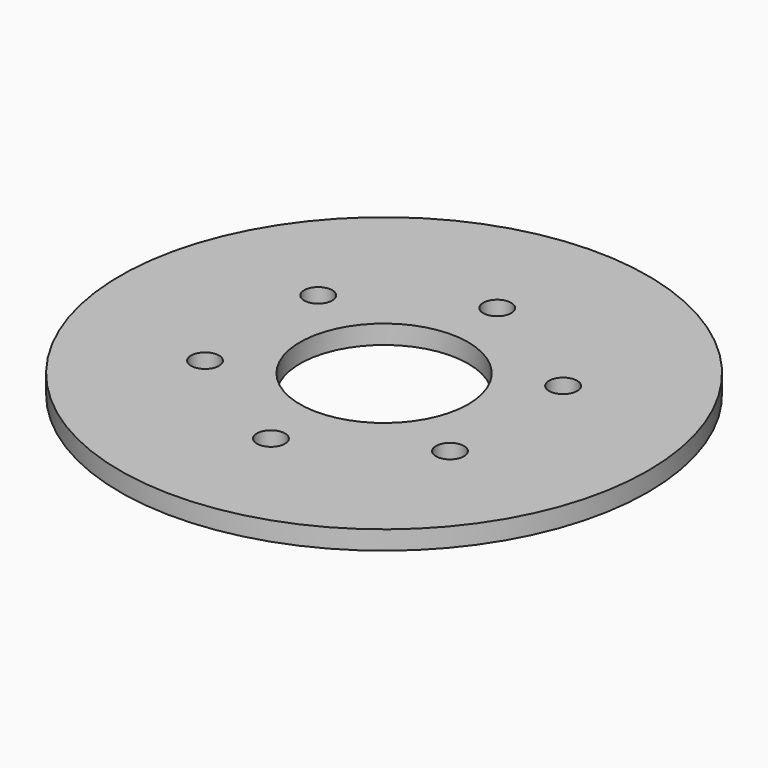
from build123d import *

# Parameters (mm, degrees)
F0_R            = 44.45
F0_R_2          = 14.1605
F1_DEPTH        = 3.175
F2_R            = 2.3622
F3_DEPTH        = 3.176
F3_COPIES_COUNT = 6


# Not quite as in the source:
# - a pattern or mirror of a feature is missing from the dataset's text; its kind, count and spacing are read off the source's solid


with BuildPart() as f1:
    # F0 (on Top) → F1 (new body)
    with BuildSketch(Plane.XY):
        Circle(F0_R)
        Circle(F0_R_2, mode=Mode.SUBTRACT)
    extrude(amount=F1_DEPTH)

    # F2 (on face) → F3 (cut, through all)
    with BuildSketch(Plane.XY.offset(3.175)):
        with Locations((0, 23.8125)):
            Circle(F2_R)
    f3 = extrude(amount=-F3_DEPTH, mode=Mode.SUBTRACT)

    # F3_copies: F3 ×6 about axis
    f3_copies_axis = Axis((0, 0, 0), (0, 0, 1))
    for i in range(1, F3_COPIES_COUNT):
        add(f3.rotate(f3_copies_axis, i * 360 / F3_COPIES_COUNT), mode=Mode.SUBTRACT)


solid = f1.part
